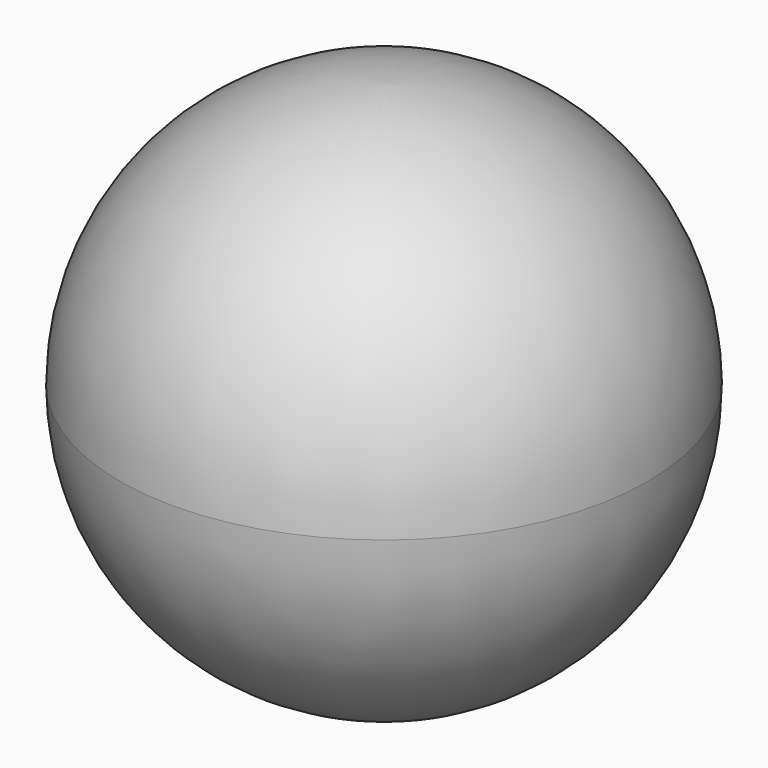
from build123d import *

# Parameters (mm, degrees)
F0_R     = 76.2
F1_DEPTH = 152.4
F2_R     = 76.19999


# Not quite as in the source:
# - a fillet or chamfer is up to 0.001 mm smaller than in the source, because OpenCascade refuses the exact size


with BuildPart() as f1:
    # F0 (on Top) → F1 (new body)
    with BuildSketch(Plane.XY):
        with Locations((-112.6874238253, 5.3689684719)):
            Circle(F0_R)
    extrude(amount=F1_DEPTH)

    # F2 (radius 76.2 in the source; OpenCascade refuses exactly that, so slightly less here)
    f2_edges = [f1.edges().sort_by_distance(p)[0] for p in [
        (-188.887424, 5.368968, 152.4),
        (-188.887424, 5.368968, 0),
    ]]
    fillet(f2_edges, radius=F2_R)


solid = f1.part
